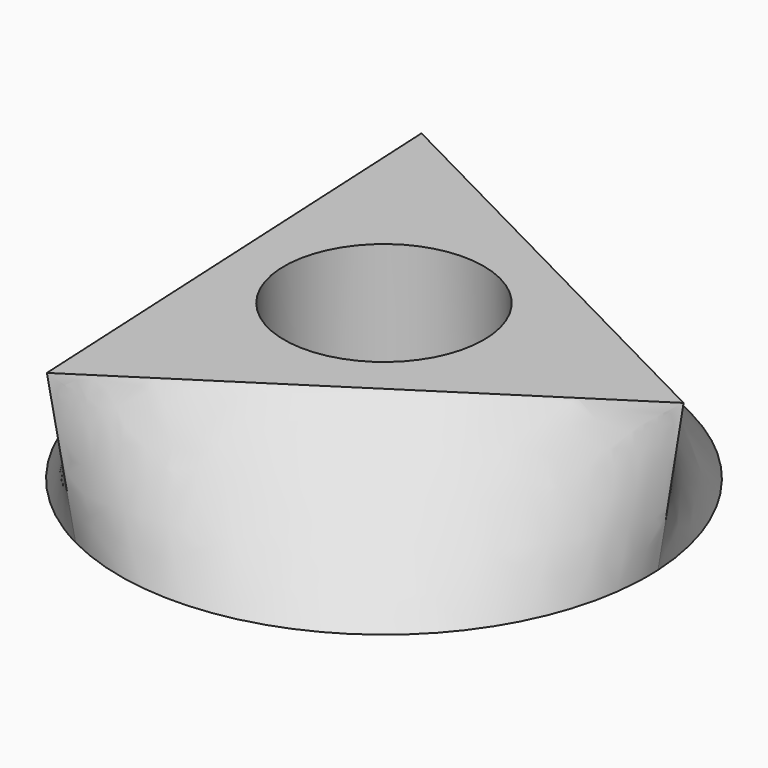
from build123d import *

# Parameters (mm, degrees)
F4_R     = 16.3873393924
F5_DEPTH = 17.78


# Not quite as in the source:
# - the arcs of a loft's sections are written as splines that run evenly, so that the points pair up as in the source's solid


with BuildPart() as f3:
    # F1 (on Top) → F3 section 0
    with BuildSketch(Plane.XY):
        with BuildLine():
            add(Edge.make_bspline(
                [(43.2906929066, 2.1420251998), (43.1660749319, 4.6605756221), (42.821117674, 7.168184659), (41.7009847964, 12.0854812551), (40.9258264748, 14.495092877), (38.9688313396, 19.1431756557), (37.7870247476, 21.3815750327), (35.0526296616, 25.6192143509), (33.5000833946, 27.6183888507), (30.071371569, 31.3168261821), (28.1952589595, 33.0160318991), (24.176410068, 36.0628920967), (22.0337358485, 37.4104995251), (17.546860581, 39.7132052837), (15.2027288233, 40.6682680536), (10.3841586143, 42.156852824), (7.9097945757, 42.6903518365), (2.9059392428, 43.3195857237), (0.3765252225, 43.4153108812), (-4.6605756221, 43.1660749319), (-7.168184659, 42.821117674), (-12.0854812551, 41.7009847964), (-14.495092877, 40.9258264748), (-19.1431756557, 38.9688313396), (-21.3815750327, 37.7870247476), (-23.5003946918, 36.4198272046)],
                knots=[0, 0, 0, 0, 0.0833333333, 0.0833333333, 0.1666666667, 0.1666666667, 0.25, 0.25, 0.3333333333, 0.3333333333, 0.4166666667, 0.4166666667, 0.5, 0.5, 0.5833333333, 0.5833333333, 0.6666666667, 0.6666666667, 0.75, 0.75, 0.8333333333, 0.8333333333, 0.9166666667, 0.9166666667, 1, 1, 1, 1], degree=3))
            add(Edge.make_bspline(
                [(-23.5003946918, 36.4198272046), (-25.6192143509, 35.0526296616), (-27.6183888507, 33.5000833946), (-31.3168261821, 30.071371569), (-33.0160318991, 28.1952589595), (-36.0628920967, 24.176410068), (-37.4104995251, 22.0337358485), (-39.7132052837, 17.546860581), (-40.6682680536, 15.2027288233), (-42.156852824, 10.3841586143), (-42.6903518365, 7.9097945757), (-43.3195857237, 2.9059392428), (-43.4153108812, 0.3765252225), (-43.1660749319, -4.6605756221), (-42.821117674, -7.168184659), (-41.7009847964, -12.0854812551), (-40.9258264748, -14.495092877), (-38.9688313396, -19.1431756557), (-37.7870247476, -21.3815750327), (-35.0526296616, -25.6192143509), (-33.5000833946, -27.6183888507), (-30.071371569, -31.3168261821), (-28.1952589595, -33.0160318991), (-24.176410068, -36.0628920967), (-22.0337358485, -37.4104995251), (-19.7902982147, -38.5618524044)],
                knots=[0, 0, 0, 0, 0.0833333333, 0.0833333333, 0.1666666667, 0.1666666667, 0.25, 0.25, 0.3333333333, 0.3333333333, 0.4166666667, 0.4166666667, 0.5, 0.5, 0.5833333333, 0.5833333333, 0.6666666667, 0.6666666667, 0.75, 0.75, 0.8333333333, 0.8333333333, 0.9166666667, 0.9166666667, 1, 1, 1, 1], degree=3))
            add(Edge.make_bspline(
                [(-19.7902982147, -38.5618524044), (-17.546860581, -39.7132052837), (-15.2027288233, -40.6682680536), (-10.3841586143, -42.156852824), (-7.9097945757, -42.6903518365), (-2.9059392428, -43.3195857237), (-0.3765252225, -43.4153108812), (4.6605756221, -43.1660749319), (7.168184659, -42.821117674), (12.0854812551, -41.7009847964), (14.495092877, -40.9258264748), (19.1431756557, -38.9688313396), (21.3815750327, -37.7870247476), (25.6192143509, -35.0526296616), (27.6183888507, -33.5000833946), (31.3168261821, -30.071371569), (33.0160318991, -28.1952589595), (36.0628920967, -24.176410068), (37.4104995251, -22.0337358485), (39.7132052837, -17.546860581), (40.6682680536, -15.2027288233), (42.156852824, -10.3841586143), (42.6903518365, -7.9097945757), (43.3195857237, -2.9059392428), (43.4153108812, -0.3765252225), (43.2906929066, 2.1420251998)],
                knots=[0, 0, 0, 0, 0.0833333333, 0.0833333333, 0.1666666667, 0.1666666667, 0.25, 0.25, 0.3333333333, 0.3333333333, 0.4166666667, 0.4166666667, 0.5, 0.5, 0.5833333333, 0.5833333333, 0.6666666667, 0.6666666667, 0.75, 0.75, 0.8333333333, 0.8333333333, 0.9166666667, 0.9166666667, 1, 1, 1, 1], degree=3))
        make_face()
    # F2 (on offset) → F3 section 1
    with BuildSketch(Plane.XY.offset(25.4)):
        Polygon((47.3345444493, 2.3421151343), (-25.6956034295, 39.8218604025), (-21.6389410198, -42.1639755368), align=None)
    loft(ruled=True)

    # F4 (on face) → F5 (cut)
    with BuildSketch(Plane.XY.offset(25.4)):
        Circle(F4_R)
    extrude(amount=-F5_DEPTH, mode=Mode.SUBTRACT)


solid = f3.part
